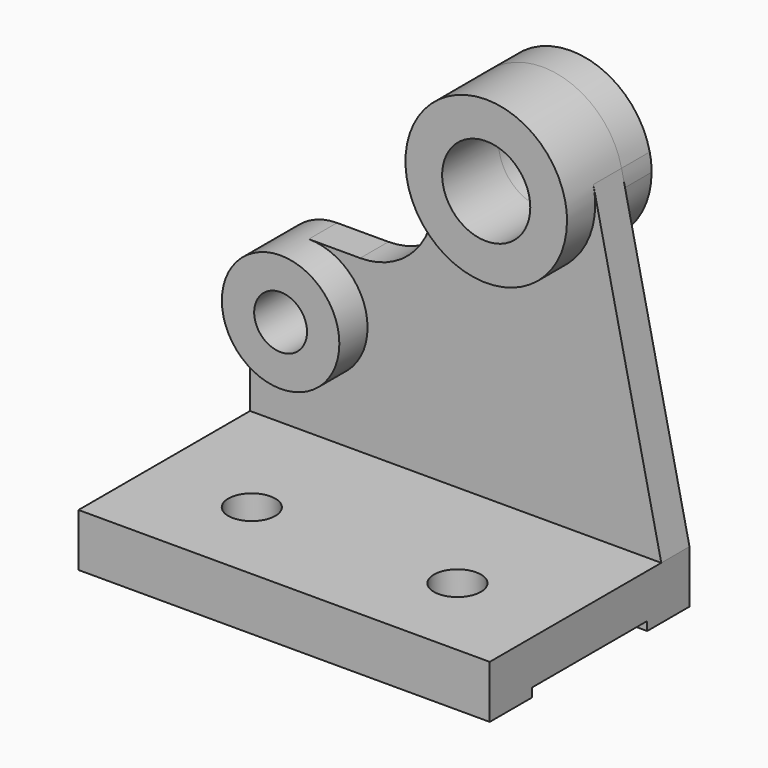
from build123d import *

# Parameters (mm, degrees)
F0_W          = 140
F0_H          = 18
F1_DEPTH      = 85
F0_R          = 9
F0_R_2        = 15
F2_DEPTH      = 12
F3_DEPTH      = 24
F4_DEPTH      = 24
F4_DEPTH_BACK = 12
F5_W          = 140
F5_H          = 49
F5_R          = 8
F6_DEPTH      = 3
F7_DEPTH      = 25


# Not quite as in the source:
# - after a boolean that leaves OpenCascade's solid faulty, fix() repairs it


with BuildPart() as f1:
    # F0 (on Front) → F1 (new body)
    with BuildSketch(Plane.XZ):
        with Locations((0, -9)):
            Rectangle(F0_W, F0_H)
    extrude(amount=F1_DEPTH)

    # F0 (on Front) → F2 (join)
    with BuildSketch(Plane.XZ):
        with BuildLine():
            Line((-70, 38), (-70, 0))
            Line((-70, 0), (70, 0))
            Line((70, 0), (46.8660884819, 105.8705442409))
            ThreePointArc((46.8660884819, 105.8705442409), (47.3410628291, 102.9523352409), (47.5, 100))
            ThreePointArc((47.5, 100), (20, 72.5), (-7.5, 100))
            Line((-7.5, 100), (-7.5, 83))
            ThreePointArc((-7.5, 83), (-14.8223304703, 65.3223304703), (-32.5, 58))
            Line((-32.5, 58), (-50, 58))
            ThreePointArc((-50, 58), (-35.8578643763, 52.1421356237), (-30, 38))
            ThreePointArc((-30, 38), (-50, 18), (-70, 38))
        make_face()
        with BuildLine():
            ThreePointArc((-50, 58), (-64.1421356237, 52.1421356237), (-70, 38))
            ThreePointArc((-70, 38), (-50, 18), (-30, 38))
            ThreePointArc((-30, 38), (-35.8578643763, 52.1421356237), (-50, 58))
        make_face()
        with Locations((-50, 38)):
            Circle(F0_R, mode=Mode.SUBTRACT)
        with BuildLine():
            ThreePointArc((47.5, 100), (47.3410628291, 102.9523352409), (46.8660884819, 105.8705442409))
            ThreePointArc((46.8660884819, 105.8705442409), (17.0476647591, 127.3410628291), (-7.5, 100))
            ThreePointArc((-7.5, 100), (20, 72.5), (47.5, 100))
        make_face()
        with Locations((20, 100)):
            Circle(F0_R_2, mode=Mode.SUBTRACT)
    extrude(amount=F2_DEPTH)

    # F0 (on Front) → F3 (join)
    with BuildSketch(Plane.XZ):
        with BuildLine():
            ThreePointArc((-50, 58), (-64.1421356237, 52.1421356237), (-70, 38))
            ThreePointArc((-70, 38), (-50, 18), (-30, 38))
            ThreePointArc((-30, 38), (-35.8578643763, 52.1421356237), (-50, 58))
        make_face()
        with Locations((-50, 38)):
            Circle(F0_R, mode=Mode.SUBTRACT)
    extrude(amount=F3_DEPTH)

    # F0 (on Front) → F4 (join, two sides)
    with BuildSketch(Plane.XZ) as f4_sk:
        with BuildLine():
            ThreePointArc((47.5, 100), (47.3410628291, 102.9523352409), (46.8660884819, 105.8705442409))
            ThreePointArc((46.8660884819, 105.8705442409), (17.0476647591, 127.3410628291), (-7.5, 100))
            ThreePointArc((-7.5, 100), (20, 72.5), (47.5, 100))
        make_face()
        with Locations((20, 100)):
            Circle(F0_R_2, mode=Mode.SUBTRACT)
    extrude(amount=F4_DEPTH)
    extrude(f4_sk.sketch, amount=-F4_DEPTH_BACK)

    add(f1.part.fix(), mode=Mode.REPLACE)

    # F5 (on face) → F6 (cut)
    with BuildSketch(Plane(origin=(0, 0, -18), x_dir=(1, 0, 0), z_dir=(0, 0, -1))):
        with Locations((0, 42.5)):
            Rectangle(F5_W, F5_H)
        with Locations((-35, 55)):
            Circle(F5_R, mode=Mode.SUBTRACT)
        with Locations((35, 55)):
            Circle(F5_R, mode=Mode.SUBTRACT)
    extrude(amount=-F6_DEPTH, mode=Mode.SUBTRACT)

    # F7 (cut): faces of the model
    f7_faces = [f1.faces().sort_by_distance(p)[0] for p in [
        (-35, -55, -18),
        (35, -55, -18),
    ]]
    extrude(f7_faces, amount=-F7_DEPTH, mode=Mode.SUBTRACT)


solid = f1.part
